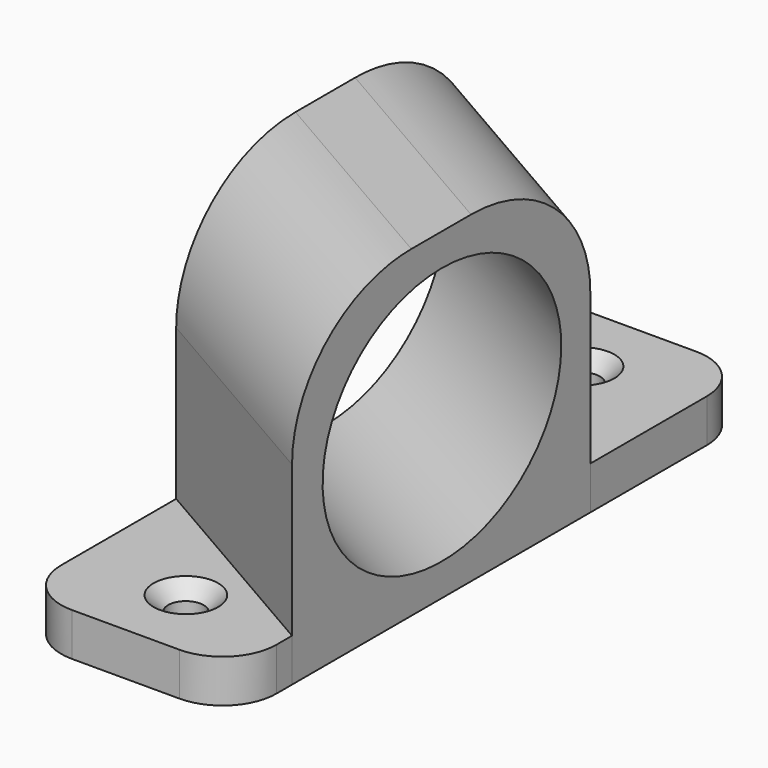
from build123d import *

# Parameters (mm, degrees)
F1_DEPTH          = 4
F2_DEPTH          = 30
F3_W              = 18.0332418531
F3_H              = 11.783156544
F4_DEPTH          = 25
F6_R              = 12
F7_DEPTH          = 25
F7_DEPTH_BACK     = 25
F8_DEPTH          = 25
F10_D             = 3.3
F10_CSINK_D       = 6
F10_CSINK_ANGLE   = 90
F10_2_D           = 3.3
F10_2_CSINK_D     = 6
F10_2_CSINK_ANGLE = 90
F11_R             = 5
F11_2_R           = 5
F12_T1_DEPTH      = 83.0940107676
F12_T3_DEPTH      = 83.0940107676


# Not quite as in the source:
# - a fillet or chamfer that OpenCascade refuses, or shapes differently, is made with other operations: its cross-section is extruded or revolved along the edge and cut away or added


with BuildPart() as f1:
    # F0 (on Top) → F1 (new body)
    with BuildSketch(Plane.XY):
        Polygon((10, 30), (-10, 30), (-10, 23.0067708135), (10, 11.4597654297), align=None)
    extrude(amount=F1_DEPTH)

    # F10 (through all)
    with Locations(Plane.XY.offset(4)):
        with Locations((0, 23.0067708135), (0, -23.0067708135)):
            CounterSinkHole(F10_D / 2, F10_CSINK_D / 2, counter_sink_angle=F10_CSINK_ANGLE)

    # F11
    f11_edges = [f1.edges().sort_by_distance(p)[0] for p in [
        (10, 30, 2),
        (-10, 30, 2),
    ]]
    fillet(f11_edges, radius=F11_R)


with BuildPart() as f1b:
    # F0 (on Top) → F1, piece 2 (new body)
    with BuildSketch(Plane.XY):
        Polygon((10, -23.1812507217), (-10, -11.6342453379), (-10, -30), (10, -30), align=None)
    extrude(amount=F1_DEPTH)

    # F10#2 (through all)
    with Locations(Plane.XY.offset(4)):
        with Locations((0, 23.0067708135), (0, -23.0067708135)):
            CounterSinkHole(F10_2_D / 2, F10_2_CSINK_D / 2, counter_sink_angle=F10_2_CSINK_ANGLE)

    # F11#2
    f11_2_edges = [f1b.edges().sort_by_distance(p)[0] for p in [
        (-10, -30, 2),
        (10, -30, 2),
    ]]
    fillet(f11_2_edges, radius=F11_2_R)


with BuildPart() as f2:
    # F0 (on Top) → F2 (new body)
    with BuildSketch(Plane.XY):
        Polygon((10, 11.4597654297), (-10, 23.0067708135), (-10, -11.6342453379), (10, -23.1812507217), align=None)
    extrude(amount=F2_DEPTH)

    # F3 (on face) → F4 (join)
    with BuildSketch(Plane(origin=(7.4622239918, 12.9249510912, 0), x_dir=(-0.8660254038, 0.5, 0), z_dir=(0.5, 0.8660254038, 0))):
        with Locations((6.0862496035, 21.4814543724)):
            Rectangle(F3_W, F3_H)
    extrude(amount=F4_DEPTH)

    # F6 (on offset) → F7 (cut, two sides)
    with BuildSketch(Plane(origin=(2.5377760082, -1.4651856615, 0), x_dir=(0.5, 0.8660254038, 0), z_dir=(0.8660254038, -0.5, 0))) as f7_sk:
        with Locations((0, 15)):
            Circle(F6_R)
    extrude(amount=-F7_DEPTH, mode=Mode.SUBTRACT)
    extrude(f7_sk.sketch, amount=F7_DEPTH_BACK, mode=Mode.SUBTRACT)

    # F8 (cut): a face of the model
    f8_faces = [f2.faces().sort_by_distance(p)[0] for p in [
        (16.25, 22.285082977, 21.4814543724),
    ]]
    extrude(f8_faces, amount=-F8_DEPTH, mode=Mode.SUBTRACT)

    # F12: fillet of radius 12 on 2 edges, made by hand

    # F12_s2 → F12_t1 (cut)
    with BuildSketch(Plane(origin=(-28.4429861053, 16.4215656844, 0), x_dir=(0, 0, 1), z_dir=(0.8660254038, -0.5, 0))):
        with BuildLine():
            ThreePointArc((18, 15.0755520165), (26.4852813742, 11.5608333907), (30, 3.0755520165))
            Line((30, 3.0755520165), (30, 15.0755520165))
            Line((30, 15.0755520165), (18, 15.0755520165))
        make_face()
    extrude(amount=F12_T1_DEPTH, mode=Mode.SUBTRACT)

    # F12_s4 → F12_t3 (cut)
    with BuildSketch(Plane(origin=(28.5185381218, -16.4651856615, 0), x_dir=(0, 0, 1), z_dir=(-0.8660254038, 0.5, 0))):
        with BuildLine():
            ThreePointArc((18, 14.9244479835), (26.4852813742, 11.4097293577), (30, 2.9244479835))
            Line((30, 2.9244479835), (30, 14.9244479835))
            Line((30, 14.9244479835), (18, 14.9244479835))
        make_face()
    extrude(amount=F12_T3_DEPTH, mode=Mode.SUBTRACT)


solid = Compound([f1.part, f1b.part, f2.part])
